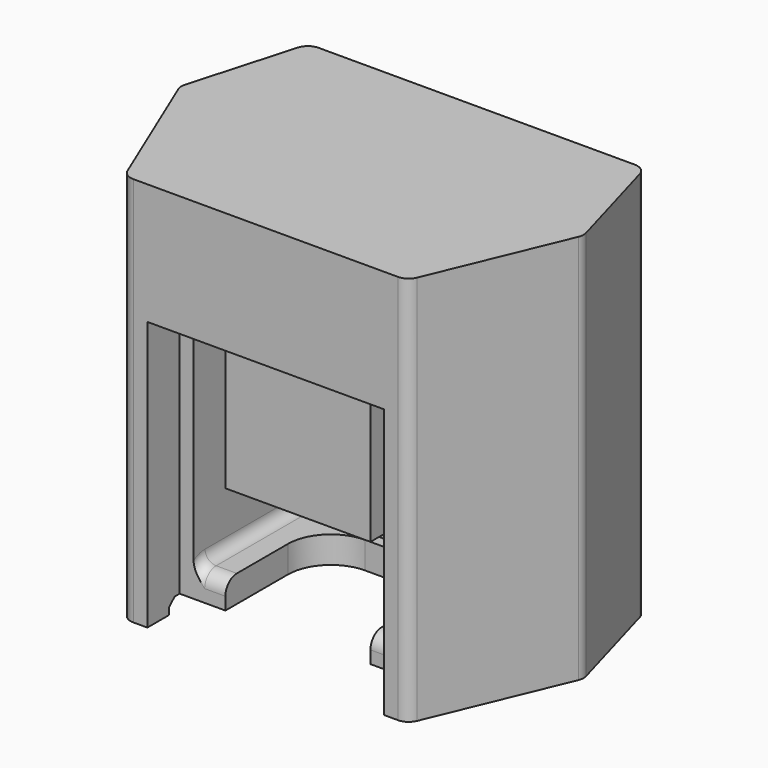
from build123d import *

# Parameters (mm, degrees)
F1_DEPTH      = 14
F3_START      = 2
F3_DEPTH      = 9.7
F4_DEPTH      = 1
F4_DEPTH_BACK = 22
F5_START      = 9.5
F5_DEPTH      = 4.5
F6_DEPTH      = 4.5
F8_DEPTH      = 0.5
F9_R          = 1.5933809512
F10_R         = 0.5311269837
F11_T1_DEPTH  = 5.3949137803
F11_T6_ANGLE  = 200.7294916834
F11_T12_ANGLE = 200.7294916834
F12_T1_DEPTH  = 1.2663530932
F12_T3_DEPTH  = 0.9362653772
F12_T5_DEPTH  = 1.4443499817
F12_T7_DEPTH  = 1.4443499817
F12_T9_DEPTH  = 0.9362653772
F12_T11_DEPTH = 1.2663530932
F12_T13_DEPTH = 16.1666666667
F12_T15_DEPTH = 16.1666666667
F12_T17_DEPTH = 15.3725307543
F12_T19_DEPTH = 16.3886999634
F12_T21_DEPTH = 16.3886999634
F12_T23_DEPTH = 15.3725307543
F13_SIZE      = 0.25


# Not quite as in the source:
# - a fillet or chamfer that OpenCascade refuses, or shapes differently, is made with other operations: its cross-section is extruded or revolved along the edge and cut away or added


with BuildPart() as f1:
    # F0 (on Top) → F1 (new body)
    with BuildSketch(Plane.XY):
        Polygon((6.25, 4.4), (0, 4.4), (-6.25, 4.4), (-7.5, 0), (-5.25, -5.4), (-4.395, -5.4), (-4.395, -3.9), (-2.695, -3.9), (-2.695, 0.6), (0, 0.6), (2.695, 0.6), (2.695, -3.9), (4.395, -3.9), (4.395, -5.4), (5.25, -5.4), (7.5, 0), align=None)
    extrude(amount=F1_DEPTH)

    # F2 (on Front) → F3 (cut)
    with BuildSketch(Plane.XZ.offset(F3_START)):
        Polygon((0, 4), (3.875, 4), (3.875, 9), (0, 9), (-3.875, 9), (-3.875, 4), align=None)
    extrude(amount=F3_DEPTH, mode=Mode.SUBTRACT)

    # F2 (on Front) → F4 (cut, two sides)
    with BuildSketch(Plane.XZ) as f4_sk:
        Polygon((-3.875, 1), (0, 1), (3.875, 1), (3.875, 4), (0, 4), (-3.875, 4), align=None)
    extrude(amount=-F4_DEPTH, mode=Mode.SUBTRACT)
    extrude(f4_sk.sketch, amount=F4_DEPTH_BACK, mode=Mode.SUBTRACT)

    # F0 (on Top) → F5 (join)
    with BuildSketch(Plane.XY.offset(F5_START)):
        Polygon((0, -5.4), (4.395, -5.4), (4.395, -3.9), (2.695, -3.9), (2.695, 0.6), (0, 0.6), (-2.695, 0.6), (-2.695, -3.9), (-4.395, -3.9), (-4.395, -5.4), align=None)
    extrude(amount=F5_DEPTH)

    # F6 (add): a face of the model
    f6_faces = [f1.faces().sort_by_distance(p)[0] for p in [
        (0, 0.6, 6.75),
    ]]
    extrude(f6_faces, amount=F6_DEPTH)

    # F7 (on face) → F8 (join)
    with BuildSketch(Plane(origin=(0, 0, 0), x_dir=(1, 0, 0), z_dir=(0, 0, -1))):
        Polygon((4.395, 5.4), (4.395, 4.4), (4.5833333333, 4.4), (6.4426875763, -0.062450183), (5.4945200146, -3.4), (-5.4945200146, -3.4), (-6.4426875763, -0.062450183), (-4.5833333333, 4.4), (-4.395, 4.4), (-4.395, 5.4), (-5.25, 5.4), (-7.5, 0), (-6.25, -4.4), (6.25, -4.4), (7.5, 0), (5.25, 5.4), align=None)
    extrude(amount=F8_DEPTH)

    # F9
    f9_edges = [f1.edges().sort_by_distance(p)[0] for p in [
        (2.695, 0.6, 0.5),
        (-2.695, 0.6, 0.5),
    ]]
    fillet(f9_edges, radius=F9_R)

    # F10
    f10_edges = [f1.edges().sort_by_distance(p)[0] for p in [
        (-3.285, -3.9, 1),
        (3.285, -3.9, 1),
    ]]
    fillet(f10_edges, radius=F10_R)

    # F11: fillet of radius 0.4104163056 on 2 edges, made by hand

    # F11_s2 → F11_t1 (join)
    with BuildSketch(Plane.XZ.offset(-2.026040764)):
        with BuildLine():
            ThreePointArc((3.4645836944, 1), (3.7547918472, 1.1202081528), (3.875, 1.4104163056))
            Line((3.875, 1.4104163056), (3.875, 1))
            Line((3.875, 1), (3.4645836944, 1))
        make_face()
        with BuildLine():
            ThreePointArc((-3.4645836944, 1), (-3.7547918472, 1.1202081528), (-3.875, 1.4104163056))
            Line((-3.875, 1.4104163056), (-3.875, 1))
            Line((-3.875, 1), (-3.4645836944, 1))
        make_face()
    extrude(amount=F11_T1_DEPTH)


with BuildPart() as f11_tool4:
    # F11_s5 → F11_t6 (revolve)
    with BuildSketch(Plane(origin=(0, -2.7915869666, -1.0564952052), x_dir=(1, 0, 0), z_dir=(0, 0.9352619639, 0.3539562952))):
        with BuildLine():
            ThreePointArc((-3.4645836944, -1.0998259262), (-3.7547918472, -0.9796177734), (-3.875, -0.6894096206))
            Line((-3.875, -0.6894096206), (-3.875, -1.0998259262))
            Line((-3.875, -1.0998259262), (-3.4645836944, -1.0998259262))
        make_face()
    revolve(axis=Axis((-3.875, -3.3688730163, 0.4688730163), (-1, 0, 0)), revolution_arc=F11_T6_ANGLE)

    split(bisect_by=Plane.XZ.offset(3.9), keep=Keep.BOTTOM)

    split(bisect_by=Plane.XY, keep=Keep.TOP)


with BuildPart() as f1_1:
    add(f1.part)

    # F11_t3: union F11_tool4
    add(f11_tool4.part)


with BuildPart() as f11_tool10:
    # F11_s11 → F11_t12 (revolve)
    with BuildSketch(Plane(origin=(0, -2.7915869666, -1.0564952052), x_dir=(1, 0, 0), z_dir=(0, 0.9352619639, 0.3539562952))):
        with BuildLine():
            ThreePointArc((3.4645836944, -1.0998259262), (3.7547918472, -0.9796177734), (3.875, -0.6894096206))
            Line((3.875, -0.6894096206), (3.875, -1.0998259262))
            Line((3.875, -1.0998259262), (3.4645836944, -1.0998259262))
        make_face()
    revolve(axis=Axis((3.875, -3.3688730163, 0.4688730163), (-1, 0, 0)), revolution_arc=F11_T12_ANGLE)

    split(bisect_by=Plane.XZ.offset(3.9), keep=Keep.BOTTOM)

    split(bisect_by=Plane.XY, keep=Keep.TOP)


with BuildPart() as f1_2:
    add(f1_1.part)

    # F11_t9: union F11_tool10
    add(f11_tool10.part)

    # F12: fillet of radius 0.5 on 12 edges, made by hand

    # F12_s2 → F12_t1 (join)
    with BuildSketch(Plane.XY.offset(-0.5)):
        with BuildLine():
            ThreePointArc((-4.395, -4.4), (-4.5790190998, -4.2919632329), (-4.7012338092, -4.1170388579))
            Line((-4.7012338092, -4.1170388579), (-4.5833333333, -4.4))
            Line((-4.5833333333, -4.4), (-4.395, -4.4))
        make_face()
    extrude(amount=F12_T1_DEPTH)

    # F12_s4 → F12_t3 (join)
    with BuildSketch(Plane.XY.offset(-0.5)):
        with BuildLine():
            ThreePointArc((-6.3755698259, -0.0986324178), (-6.4131614706, 0.0641941432), (-6.3949990431, 0.2303138196))
            Line((-6.3949990431, 0.2303138196), (-6.4426875763, 0.062450183))
            Line((-6.4426875763, 0.062450183), (-6.3755698259, -0.0986324178))
        make_face()
    extrude(amount=F12_T3_DEPTH)

    # F12_s6 → F12_t5 (join)
    with BuildSketch(Plane.XY.offset(-0.5)):
        with BuildLine():
            ThreePointArc((-5.5977477007, 3.0366385451), (-5.4181773738, 3.2989481624), (-5.1167800219, 3.4))
            Line((-5.1167800219, 3.4), (-5.4945200146, 3.4))
            Line((-5.4945200146, 3.4), (-5.5977477007, 3.0366385451))
        make_face()
    extrude(amount=F12_T5_DEPTH)

    # F12_s8 → F12_t7 (join)
    with BuildSketch(Plane.XY.offset(-0.5)):
        with BuildLine():
            ThreePointArc((5.1167800219, 3.4), (5.4181773738, 3.2989481624), (5.5977477007, 3.0366385451))
            Line((5.5977477007, 3.0366385451), (5.4945200146, 3.4))
            Line((5.4945200146, 3.4), (5.1167800219, 3.4))
        make_face()
    extrude(amount=F12_T7_DEPTH)

    # F12_s10 → F12_t9 (join)
    with BuildSketch(Plane.XY.offset(-0.5)):
        with BuildLine():
            ThreePointArc((6.3949990431, 0.2303138196), (6.4131614706, 0.0641941432), (6.3755698259, -0.0986324178))
            Line((6.3755698259, -0.0986324178), (6.4426875763, 0.062450183))
            Line((6.4426875763, 0.062450183), (6.3949990431, 0.2303138196))
        make_face()
    extrude(amount=F12_T9_DEPTH)

    # F12_s12 → F12_t11 (join)
    with BuildSketch(Plane.XY.offset(-0.5)):
        with BuildLine():
            ThreePointArc((4.7012338092, -4.1170388579), (4.5790190998, -4.2919632329), (4.395, -4.4))
            Line((4.395, -4.4), (4.5833333333, -4.4))
            Line((4.5833333333, -4.4), (4.7012338092, -4.1170388579))
        make_face()
    extrude(amount=F12_T11_DEPTH)

    # F12_s14 → F12_t13 (cut)
    with BuildSketch(Plane.XY.offset(-1.3333333333)):
        with BuildLine():
            ThreePointArc((-4.9166666667, -5.4), (-5.1940167648, -5.3160251472), (-5.3782051282, -5.0923076923))
            Line((-5.3782051282, -5.0923076923), (-5.25, -5.4))
            Line((-5.25, -5.4), (-4.9166666667, -5.4))
        make_face()
    extrude(amount=F12_T13_DEPTH, mode=Mode.SUBTRACT)

    # F12_s16 → F12_t15 (cut)
    with BuildSketch(Plane.XY.offset(-1.3333333333)):
        with BuildLine():
            ThreePointArc((4.9166666667, -5.4), (5.1940167648, -5.3160251472), (5.3782051282, -5.0923076923))
            Line((5.3782051282, -5.0923076923), (5.25, -5.4))
            Line((5.25, -5.4), (4.9166666667, -5.4))
        make_face()
    extrude(amount=F12_T15_DEPTH, mode=Mode.SUBTRACT)

    # F12_s18 → F12_t17 (cut)
    with BuildSketch(Plane.XY.offset(-0.9362653772)):
        with BuildLine():
            ThreePointArc((7.4328822497, -0.1610826008), (7.4704738943, 0.0017439601), (7.4523114669, 0.1678636366))
            Line((7.4523114669, 0.1678636366), (7.5, 0))
            Line((7.5, 0), (7.4328822497, -0.1610826008))
        make_face()
    extrude(amount=F12_T17_DEPTH, mode=Mode.SUBTRACT)

    # F12_s20 → F12_t19 (cut)
    with BuildSketch(Plane.XY.offset(-1.4443499817)):
        with BuildLine():
            ThreePointArc((6.3532276861, 4.0366385451), (6.1736573592, 4.2989481624), (5.8722600073, 4.4))
            Line((5.8722600073, 4.4), (6.25, 4.4))
            Line((6.25, 4.4), (6.3532276861, 4.0366385451))
        make_face()
    extrude(amount=F12_T19_DEPTH, mode=Mode.SUBTRACT)

    # F12_s22 → F12_t21 (cut)
    with BuildSketch(Plane.XY.offset(-1.4443499817)):
        with BuildLine():
            ThreePointArc((-5.8722600073, 4.4), (-6.1736573592, 4.2989481624), (-6.3532276861, 4.0366385451))
            Line((-6.3532276861, 4.0366385451), (-6.25, 4.4))
            Line((-6.25, 4.4), (-5.8722600073, 4.4))
        make_face()
    extrude(amount=F12_T21_DEPTH, mode=Mode.SUBTRACT)

    # F12_s24 → F12_t23 (cut)
    with BuildSketch(Plane.XY.offset(-0.9362653772)):
        with BuildLine():
            ThreePointArc((-7.4523114669, 0.1678636366), (-7.4704738943, 0.0017439601), (-7.4328822497, -0.1610826008))
            Line((-7.4328822497, -0.1610826008), (-7.5, 0))
            Line((-7.5, 0), (-7.4523114669, 0.1678636366))
        make_face()
    extrude(amount=F12_T23_DEPTH, mode=Mode.SUBTRACT)

    # F13
    f13_edges = [f1_2.edges().sort_by_distance(p)[0] for p in [
        (-5.996373, 1.633476, 0),
        (-5.418177, 3.298948, 0),
        (-6.413161, 0.064194, 0),
        (-5.538402, -2.107836, 0),
        (-4.579019, -4.291963, 0),
        (4.579019, -4.291963, 0),
        (5.538402, -2.107836, 0),
        (6.413161, 0.064194, 0),
        (5.996373, 1.633476, 0),
        (5.418177, 3.298948, 0),
        (0, 3.4, 0),
    ]]
    chamfer(f13_edges, length=F13_SIZE)


solid = f1_2.part
